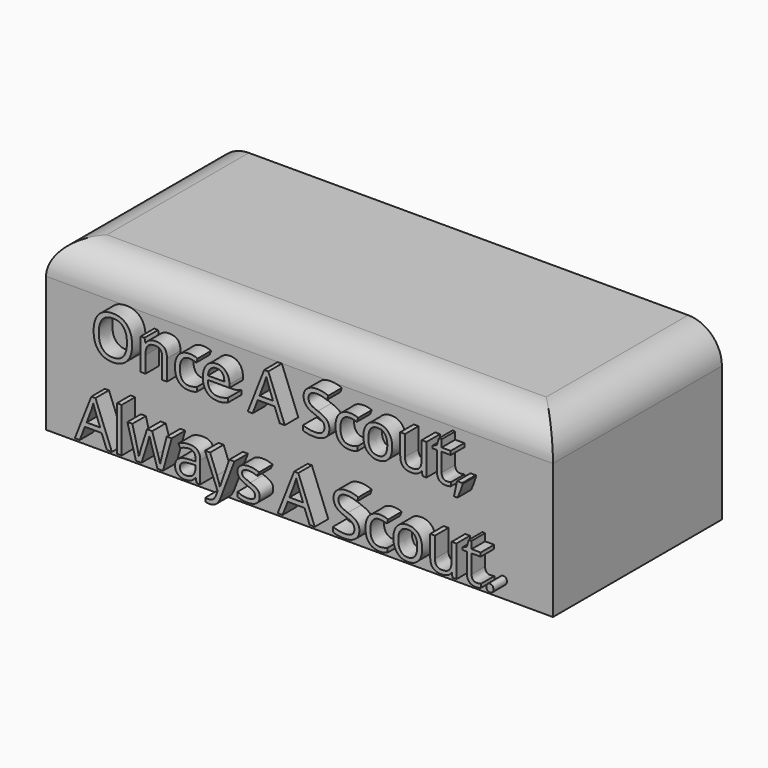
from build123d import *

# Parameters (mm, degrees)
F0_W         = 76.2
F0_H         = 31.75
F1_DEPTH     = 25.4
F2_R         = 5.08
F3_TEXT_SIZE = 8.8125596322
F4_DEPTH     = 2.54


# Not quite as in the source:
# - Text() gives the source's letters only with a copy of the font that has no kerning and outlines rounded to 1/6400 em; it was checked with that copy


with BuildPart() as f1:
    # F0 (on Top) → F1 (new body)
    with BuildSketch(Plane.XY):
        with Locations((-38.1, 15.875)):
            Rectangle(F0_W, F0_H)
    extrude(amount=F1_DEPTH)

    # F2
    f2_edges = [f1.edges().sort_by_distance(p)[0] for p in [
        (-38.1, 0, 25.4),
        (-76.2, 15.875, 25.4),
        (0, 15.875, 25.4),
    ]]
    fillet(f2_edges, radius=F2_R)

    # F3 (on face) → F4 (join)
    with BuildSketch(Plane.XZ):
        with Locations((-67.5601114581, 13.9749570648)):
            Text('Once A Scout,', F3_TEXT_SIZE, font='Open Sans', text_align=(TextAlign.LEFT, TextAlign.BOTTOM))
        with Locations((-69.85, 1.989875965)):
            Text('Always A Scout.', F3_TEXT_SIZE, font='Open Sans', text_align=(TextAlign.LEFT, TextAlign.BOTTOM))
    extrude(amount=F4_DEPTH)


solid = f1.part
